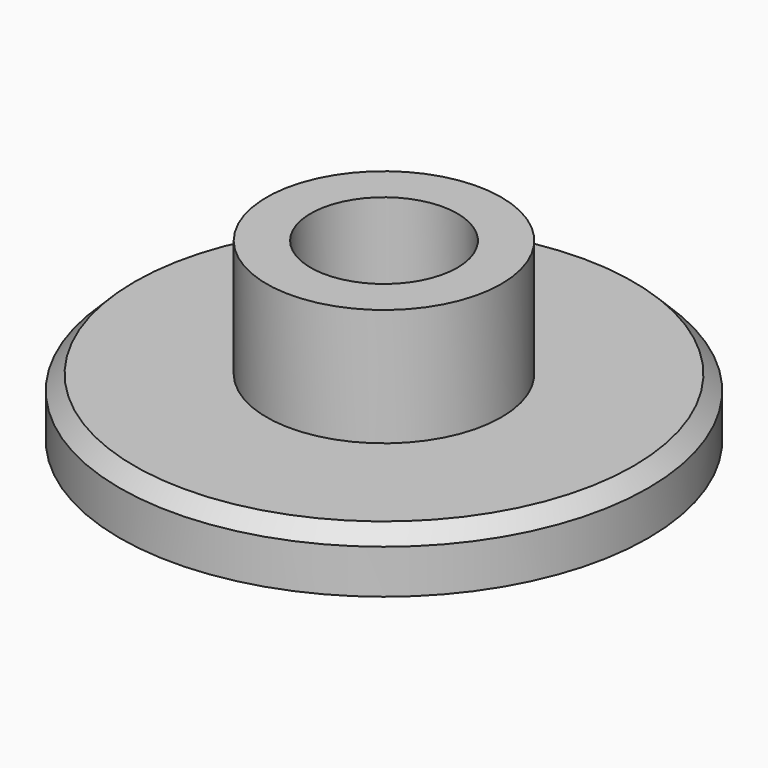
from build123d import *

# Parameters (mm, degrees)
F0_R     = 9
F1_DEPTH = 2
F2_R     = 4
F3_DEPTH = 4
F4_R     = 2.5
F5_DEPTH = 3
F6_SIZE  = 0.5
F8_DEPTH = 1.5


with BuildPart() as f1:
    # F0 (on Top) → F1 (new body)
    with BuildSketch(Plane.XY):
        Circle(F0_R)
    extrude(amount=F1_DEPTH)

    # F2 (on face) → F3 (join)
    with BuildSketch(Plane.XY.offset(2)):
        Circle(F2_R)
    extrude(amount=F3_DEPTH)

    # F4 (on face) → F5 (cut)
    with BuildSketch(Plane.XY.offset(6)):
        Circle(F4_R)
    extrude(amount=-F5_DEPTH, mode=Mode.SUBTRACT)

    # F6
    f6_edges = [f1.edges().sort_by_distance(p)[0] for p in [
        (-9, 0, 2),
    ]]
    chamfer(f6_edges, length=F6_SIZE)

    # F7 (on face) → F8 (cut)
    with BuildSketch(Plane(origin=(0, 0, 0), x_dir=(1, 0, 0), z_dir=(0, 0, -1))):
        Polygon((-0.031379, 5.948377), (-0.235333, 5.919157), (-0.372759, 5.868757), (-0.500818, 5.801363), (-0.64831, 5.683569), (-0.711513, 5.643549), (-0.766303, 5.595223), (-0.884297, 5.389084), (-0.972792, 2.355883), (-1.91674, 3.298237), (-2.464657, 3.842872), (-2.74588, 4.106761), (-3.037677, 4.358384), (-3.197437, 4.424921), (-3.362159, 4.476179), (-3.5244, 4.487041), (-3.686641, 4.476179), (-4.011123, 4.358384), (-4.276609, 4.122796), (-4.349034, 4.030994), (-4.401972, 3.928468), (-4.483097, 3.710516), (-4.483097, 3.357134), (-4.394602, 3.092097), (-4.24711, 2.885957), (-3.303163, 1.914155), (-2.359215, 0.971802), (-5.220556, 0.942353), (-5.397547, 0.883456), (-5.427045, 0.854008), (-5.556038, 0.793243), (-5.614945, 0.756011), (-5.663032, 0.706765), (-5.840022, 0.471176), (-5.958016, 0.117794), (-5.958016, -0.058897), (-5.940408, -0.209293), (-5.899019, -0.353383), (-5.843566, -0.461413), (-5.781025, -0.559523), (-5.655249, -0.699811), (-5.51554, -0.82456), (-5.220556, -0.942354), (-5.075648, -0.968558), (-4.928112, -0.97628), (-4.630589, -0.971802), (-4.188114, -0.971802), (-2.359215, -0.971802), (-2.368134, -1.005446), (-2.388713, -1.030699), (-3.332661, -1.973053), (-4.276609, -2.915406), (-4.34313, -2.999393), (-4.394602, -3.092097), (-4.419005, -3.155066), (-4.453599, -3.209892), (-4.476923, -3.415726), (-4.483097, -3.622171), (-4.464349, -3.757662), (-4.424101, -3.887208), (-4.374765, -3.997645), (-4.306107, -4.093348), (-4.188114, -4.240591), (-4.103985, -4.307), (-4.011123, -4.358385), (-3.71614, -4.476179), (-3.391658, -4.476179), (-3.067176, -4.387833), (-2.890186, -4.240591), (-1.946238, -3.298237), (-1.00229, -2.355884), (-0.884297, -5.418533), (-0.8253, -5.506878), (-0.699524, -5.647167), (-0.559815, -5.771915), (-0.503448, -5.807594), (-0.441821, -5.830812), (-0.341941, -5.885287), (-0.235333, -5.919158), (0.089149, -5.948606), (0.384133, -5.889709), (0.708615, -5.654121), (0.754319, -5.61094), (0.790702, -5.558969), (0.856107, -5.447981), (0.9741, -5.094599), (0.9741, -4.417282), (0.9741, -2.591472), (0.971489, -2.477691), (0.979459, -2.426523), (1.003599, -2.385332), (1.947546, -3.327686), (2.891494, -4.270039), (3.122896, -4.385014), (3.363468, -4.476179), (3.68795, -4.476179), (3.805943, -4.446731), (3.94337, -4.39633), (4.071429, -4.328936), (4.218921, -4.211142), (4.425409, -3.916657), (4.513904, -3.474929), (4.444862, -3.229831), (4.398065, -3.113042), (4.336914, -3.003752), (4.300041, -2.947904), (4.277917, -2.885958), (3.33397, -1.943604), (2.390022, -1.001251), (2.41952, -0.971802), (2.861996, -0.971802), (4.690894, -0.971802), (4.972609, -0.968567), (5.251363, -0.942354), (5.280862, -0.912905), (5.546347, -0.82456), (5.723337, -0.61842), (5.839817, -0.478169), (5.883167, -0.404005), (5.900327, -0.323934), (5.934856, -0.237188), (5.954737, -0.147151), (5.958016, 0.039233), (5.925076, 0.228087), (5.870829, 0.412279), (5.7562, 0.594983), (5.685681, 0.672036), (5.605344, 0.736213), (5.428354, 0.883456), (5.192367, 0.942353), (4.838344, 0.987761), (4.482387, 1.011028), (3.766457, 1.011578), (3.048146, 0.984877), (2.331025, 0.971802), (3.274973, 1.914155), (4.218921, 2.856509), (4.337268, 2.979647), (4.379451, 3.047229), (4.395911, 3.121546), (4.454907, 3.209891), (4.513904, 3.504377), (4.444233, 3.827854), (4.386266, 3.98061), (4.307416, 4.122796), (4.04193, 4.358384), (3.717448, 4.476179), (3.555567, 4.481563), (3.392966, 4.476179), (3.215976, 4.44673), (3.186478, 4.417282), (3.038986, 4.358384), (2.944209, 4.294123), (2.861996, 4.211142), (1.918048, 3.268788), (0.9741, 2.326435), (0.9741, 3.092097), (0.9741, 4.947355), (0.94889, 5.186814), (0.885605, 5.418532), (0.649618, 5.713018), (0.576669, 5.769819), (0.540299, 5.792295), (0.502126, 5.801363), (0.468426, 5.810267), (0.44313, 5.830812), (0.313926, 5.898818), (0.177644, 5.948606), align=None)
    extrude(amount=-F8_DEPTH, mode=Mode.SUBTRACT)


solid = f1.part
